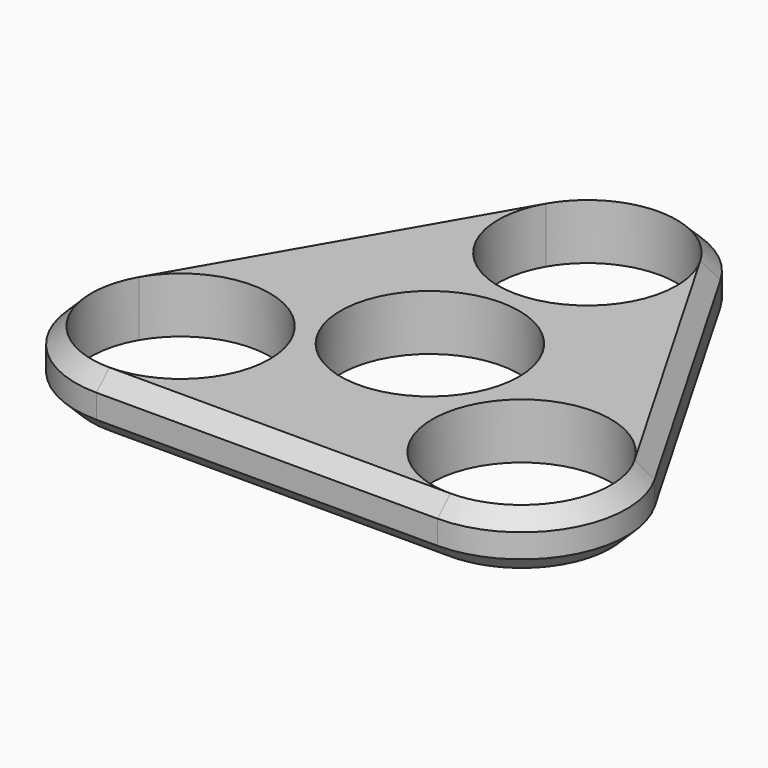
from build123d import *

# Parameters (mm, degrees)
F0_R     = 11.25
F1_DEPTH = 7
F2_SIZE  = 1.99999


# Not quite as in the source:
# - a fillet or chamfer is up to 0.001 mm smaller than in the source, because OpenCascade refuses the exact size
# - a feature names something its author has since deleted; it is built from what else it names


with BuildPart() as f1:
    # F0 (on Top) → F1 (new body)
    with BuildSketch(Plane.XY):
        with BuildLine():
            ThreePointArc((32.9748366001, -13.25), (44.4496732003, -6.625), (44.4496732003, 6.625))
            ThreePointArc((44.4496732003, 6.625), (35.3296022004, 13.0390789156), (24.5421176937, 10.2201639833))
            ThreePointArc((24.5421176937, 10.2201639833), (22.9496732003, 19.0380307876), (16.1093987873, 24.8260615752))
            ThreePointArc((16.1093987873, 24.8260615752), (23.9443929832, 32.7588397347), (22.9496732003, 43.8640923627))
            ThreePointArc((22.9496732003, 43.8640923627), (11.4748366001, 50.4890923627), (0, 43.8640923627))
            ThreePointArc((0, 43.8640923627), (-1.6185408213, 35.2078445445), (2.5465871703, 27.4488491524))
            ThreePointArc((2.5465871703, 27.4488491524), (4.5677953806, 25.931781383), (6.840274413, 24.8260615752))
            ThreePointArc((6.840274413, 24.8260615752), (0, 19.0380307876), (-1.5924444934, 10.2201639833))
            ThreePointArc((-1.5924444934, 10.2201639833), (-12.3799290001, 13.0390789156), (-21.5, 6.625))
            ThreePointArc((-21.5, 6.625), (-21.5, -6.625), (-10.0251633999, -13.25))
            ThreePointArc((-10.0251633999, -13.25), (0.0896273829, -8.5588262876), (3.0421176937, 2.1928668043))
            ThreePointArc((3.0421176937, 2.1928668043), (11.4748366001, -0.8369692124), (19.9075555066, 2.1928668043))
            ThreePointArc((19.9075555066, 2.1928668043), (22.8600458174, -8.5588262876), (32.9748366001, -13.25))
        make_face()
        with BuildLine():
            ThreePointArc((-19.7679491924, 5.625), (-7.1134491425, 10.8666655458), (1.2248366001, 0))
            ThreePointArc((1.2248366001, 0), (-2.0702121115, -7.9549512883), (-10.0251633999, -11.25))
            ThreePointArc((-10.0251633999, -11.25), (-19.7679491924, -5.625), (-19.7679491924, 5.625))
        make_face(mode=Mode.SUBTRACT)
        with BuildLine():
            ThreePointArc((44.2248366001, 0), (40.9297878885, -7.9549512883), (32.9748366001, -11.25))
            ThreePointArc((32.9748366001, -11.25), (23.2320508076, 5.625), (42.7176223927, 5.625))
            ThreePointArc((42.7176223927, 5.625), (43.8415021459, 2.9117142574), (44.2248366001, 0))
        make_face(mode=Mode.SUBTRACT)
        with Locations((11.4748366001, 12.4130307876)):
            Circle(F0_R, mode=Mode.SUBTRACT)
        with BuildLine():
            ThreePointArc((1.7320508076, 42.8640923627), (14.3865508575, 48.1057579085), (22.7248366001, 37.2390923627))
            ThreePointArc((22.7248366001, 37.2390923627), (8.5631223427, 26.372426817), (1.7320508076, 42.8640923627))
        make_face(mode=Mode.SUBTRACT)
        with BuildLine():
            ThreePointArc((2.5465871703, 27.4488491524), (-1.6185408213, 35.2078445445), (0, 43.8640923627))
            Line((0, 43.8640923627), (-21.5, 6.625))
            ThreePointArc((-21.5, 6.625), (-12.3799290001, 13.0390789156), (-1.5924444934, 10.2201639833))
            ThreePointArc((-1.5924444934, 10.2201639833), (0, 19.0380307876), (6.840274413, 24.8260615752))
            ThreePointArc((6.840274413, 24.8260615752), (4.5677953806, 25.931781383), (2.5465871703, 27.4488491524))
        make_face()
        with BuildLine():
            ThreePointArc((24.5421176937, 10.2201639833), (35.3296022004, 13.0390789156), (44.4496732003, 6.625))
            Line((44.4496732003, 6.625), (22.9496732003, 43.8640923627))
            ThreePointArc((22.9496732003, 43.8640923627), (23.9443929832, 32.7588397347), (16.1093987873, 24.8260615752))
            ThreePointArc((16.1093987873, 24.8260615752), (22.9496732003, 19.0380307876), (24.5421176937, 10.2201639833))
        make_face()
        with BuildLine():
            Line((-10.0251633999, -13.25), (32.9748366001, -13.25))
            ThreePointArc((32.9748366001, -13.25), (22.8600458174, -8.5588262876), (19.9075555066, 2.1928668043))
            ThreePointArc((19.9075555066, 2.1928668043), (11.4748366001, -0.8369692124), (3.0421176937, 2.1928668043))
            ThreePointArc((3.0421176937, 2.1928668043), (0.0896273829, -8.5588262876), (-10.0251633999, -13.25))
        make_face()
    extrude(amount=F1_DEPTH)

    # F2 (size 2 in the source; OpenCascade refuses exactly that, so slightly less here)
    f2_edges = [f1.edges().sort_by_distance(p)[0] for p in [
        (33.699673, 25.244546, 0),
        (44.449673, -6.625, 0),
        (11.474837, -13.25, 0),
        (-21.5, -6.625, 0),
        (-10.75, 25.244546, 0),
        (11.474837, 50.489092, 0),
        (-10.75, 25.244546, 7),
    ]]
    chamfer(f2_edges, length=F2_SIZE)


solid = f1.part
